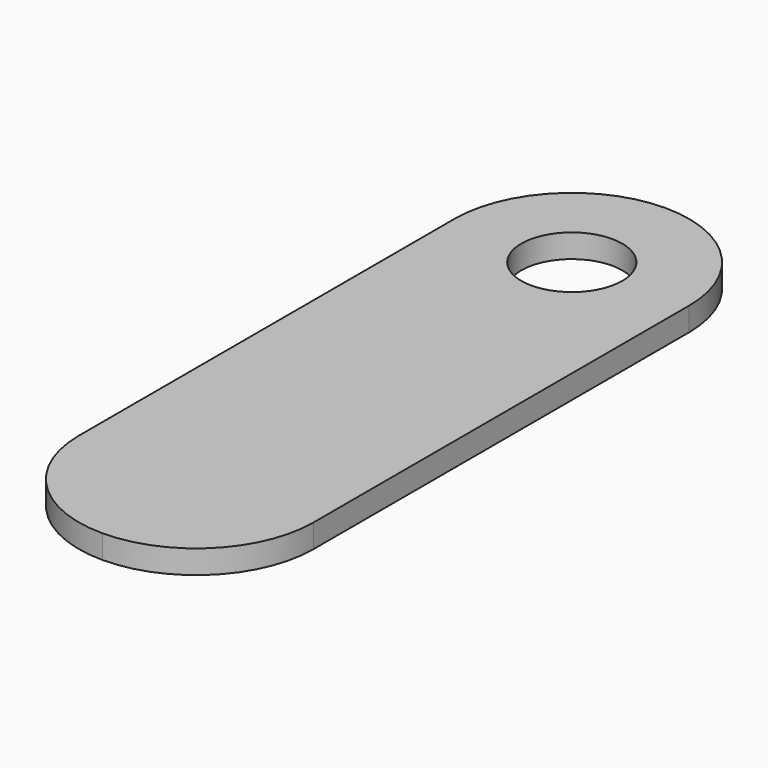
from build123d import *

# Parameters (mm, degrees)
F0_W     = 23.25
F0_H     = 69.75
F0_R     = 5
F1_DEPTH = 2.33
F2_R     = 11.62499


# Not quite as in the source:
# - a fillet or chamfer is up to 0.001 mm smaller than in the source, because OpenCascade refuses the exact size


with BuildPart() as f1:
    # F0 (on Top) → F1 (new body)
    with BuildSketch(Plane.XY):
        with Locations((11.625, 34.875)):
            Rectangle(F0_W, F0_H)
        with Locations((11.625, 58.125)):
            Circle(F0_R, mode=Mode.SUBTRACT)
    extrude(amount=F1_DEPTH)

    # F2 (radius 11.625 in the source; OpenCascade refuses exactly that, so slightly less here)
    f2_edges = [f1.edges().sort_by_distance(p)[0] for p in [
        (23.25, 0, 1.165),
        (0, 0, 1.165),
        (0, 69.75, 1.165),
        (23.25, 69.75, 1.165),
    ]]
    fillet(f2_edges, radius=F2_R)


solid = f1.part
